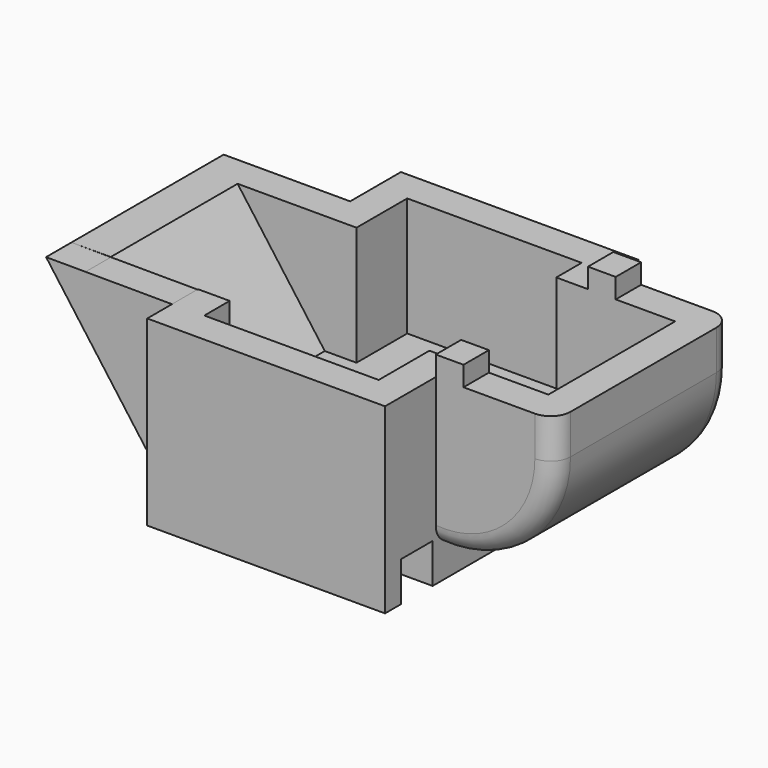
from build123d import *

# Parameters (mm, degrees)
F0_W      = 60
F0_H      = 80
F2_DEPTH  = 46
F1_W      = 30
F1_H      = 10
F3_DEPTH  = 10
F4_W      = 44
F4_H      = 64
F5_DEPTH  = 30
F6_W      = 8
F6_H      = 48
F7_DEPTH  = 30
F8_W      = 22
F8_H      = 30
F8_W_2    = 8
F9_DEPTH  = 8
F10_R     = 20
F12_DEPTH = 8
F14_DEPTH = 40
F15_R     = 5
F17_DEPTH = 8
F18_R     = 5
F19_W     = 7
F19_H     = 8
F20_DEPTH = 5
F21_W     = 22
F21_H     = 30
F21_W_2   = 8
F22_DEPTH = 8
F23_SIZE2 = 29.99999
F23_SIZE  = 21.99999
F25_DEPTH = 8
F27_DEPTH = 40
F29_DEPTH = 8


# Not quite as in the source:
# - a fillet or chamfer is up to 0.001 mm smaller than in the source, because OpenCascade refuses the exact size


with BuildPart() as f2:
    # F0 (on Top) → F2 (new body)
    with BuildSketch(Plane.XY):
        Rectangle(F0_W, F0_H)
    extrude(amount=F2_DEPTH)

    # F1 (on face) → F3 (cut)
    with BuildSketch(Plane.XY):
        with Locations((-15, 30)):
            Rectangle(F1_W, F1_H)
        with Locations((15, -30)):
            Rectangle(F1_W, F1_H)
    extrude(amount=F3_DEPTH, mode=Mode.SUBTRACT)

    # F4 (on face) → F5 (cut)
    with BuildSketch(Plane.XY.offset(46)):
        Rectangle(F4_W, F4_H)
    extrude(amount=-F5_DEPTH, mode=Mode.SUBTRACT)

    # F6 (on face) → F7 (cut, through all)
    with BuildSketch(Plane.XY.offset(46)):
        with Locations((-26, 0)):
            Rectangle(F6_W, F6_H)
        with Locations((26, 0)):
            Rectangle(F6_W, F6_H)
    extrude(amount=-F7_DEPTH, mode=Mode.SUBTRACT)

    # F8 (on face) → F9 (join)
    with BuildSketch(Plane(origin=(0, -24, 0), x_dir=(-1, 0, 0), z_dir=(0, 1, 0))):
        with Locations((-41, 31)):
            Rectangle(F8_W, F8_H)
        with Locations((-26, 31)):
            Rectangle(F8_W_2, F8_H)
    extrude(amount=F9_DEPTH)

    # F10
    f10_edges = [f2.edges().sort_by_distance(p)[0] for p in [
        (52, -20, 16),
    ]]
    fillet(f10_edges, radius=F10_R)

    # F11 (on face) → F12 (join, through all)
    with BuildSketch(Plane(origin=(0, -16, 0), x_dir=(-1, 0, 0), z_dir=(0, 1, 0))):
        with BuildLine():
            ThreePointArc((-58.1533936612, 46), (-59.5344785906, 41.08453427), (-60, 36))
            ThreePointArc((-60, 36), (-51.7989898732, 16.2010101268), (-32, 8))
            Line((-32, 8), (-32, 16))
            ThreePointArc((-32, 16), (-46.1421356237, 21.8578643763), (-52, 36))
            Line((-52, 36), (-52, 46))
            Line((-52, 46), (-58.1533936612, 46))
        make_face()
        with BuildLine():
            Line((-60, 46), (-60, 36))
            ThreePointArc((-60, 36), (-59.5344785906, 41.08453427), (-58.1533936612, 46))
            Line((-58.1533936612, 46), (-60, 46))
        make_face()
        with BuildLine():
            Line((-32, 16), (-32, 8))
            ThreePointArc((-32, 8), (-30.999360817, 8.0178856906), (-30, 8.0715199125))
            Line((-30, 8.0715199125), (-30, 16))
            Line((-30, 16), (-32, 16))
        make_face()
    extrude(amount=-F12_DEPTH)

    # F13 (on face) → F14 (join, through all)
    with BuildSketch(Plane(origin=(0, -16, 0), x_dir=(-1, 0, 0), z_dir=(0, 1, 0))):
        with BuildLine():
            ThreePointArc((-58.1533936612, 46), (-59.5344785906, 41.08453427), (-60, 36))
            Line((-60, 36), (-52, 36))
            Line((-52, 36), (-52, 46))
            Line((-52, 46), (-58.1533936612, 46))
        make_face()
        with BuildLine():
            Line((-60, 46), (-60, 36))
            ThreePointArc((-60, 36), (-59.5344785906, 41.08453427), (-58.1533936612, 46))
            Line((-58.1533936612, 46), (-60, 46))
        make_face()
        with BuildLine():
            Line((-52, 36), (-60, 36))
            ThreePointArc((-60, 36), (-51.7989898732, 16.2010101268), (-32, 8))
            Line((-32, 8), (-32, 16))
            ThreePointArc((-32, 16), (-46.1421356237, 21.8578643763), (-52, 36))
        make_face()
        with BuildLine():
            Line((-32, 16), (-32, 8))
            ThreePointArc((-32, 8), (-30.999360817, 8.0178856906), (-30, 8.0715199125))
            Line((-30, 8.0715199125), (-30, 16))
            Line((-30, 16), (-32, 16))
        make_face()
    extrude(amount=F14_DEPTH)

    # F15
    f15_edges = [f2.edges().sort_by_distance(p)[0] for p in [
        (51.078784, -24, 15.506098),
    ]]
    fillet(f15_edges, radius=F15_R)

    # F16 (on face) → F17 (join)
    with BuildSketch(Plane(origin=(0, 24, 0), x_dir=(-1, 0, 0), z_dir=(0, 1, 0))):
        with BuildLine():
            ThreePointArc((-30, 8.0715199125), (-30.999360817, 8.0178856906), (-32, 8))
            Line((-32, 8), (-30, 8))
            Line((-30, 8), (-30, 8.0715199125))
        make_face()
        with BuildLine():
            Line((-30, 16), (-32, 16))
            Line((-32, 16), (-32, 8))
            ThreePointArc((-32, 8), (-30.999360817, 8.0178856906), (-30, 8.0715199125))
            Line((-30, 8.0715199125), (-30, 16))
        make_face()
        with BuildLine():
            ThreePointArc((-32, 16), (-46.1421356237, 21.8578643763), (-52, 36))
            Line((-52, 36), (-60, 36))
            ThreePointArc((-60, 36), (-51.7989898732, 16.2010101268), (-32, 8))
            Line((-32, 8), (-32, 16))
        make_face()
        with BuildLine():
            Line((-60, 46), (-60, 36))
            ThreePointArc((-60, 36), (-59.5344785906, 41.08453427), (-58.1533936612, 46))
            Line((-58.1533936612, 46), (-60, 46))
        make_face()
        with BuildLine():
            Line((-60, 36), (-52, 36))
            Line((-52, 36), (-52, 46))
            Line((-52, 46), (-58.1533936612, 46))
            ThreePointArc((-58.1533936612, 46), (-59.5344785906, 41.08453427), (-60, 36))
        make_face()
        with BuildLine():
            ThreePointArc((-30, 16.1002512579), (-30.9987444988, 16.0250785378), (-32, 16))
            Line((-32, 16), (-30, 16))
            Line((-30, 16), (-30, 16.1002512579))
        make_face()
        with BuildLine():
            ThreePointArc((-49.3205080757, 46), (-51.3185165258, 41.1763809021), (-52, 36))
            ThreePointArc((-52, 36), (-46.1421356237, 21.8578643763), (-32, 16))
            ThreePointArc((-32, 16), (-30.9987444988, 16.0250785378), (-30, 16.1002512579))
            Line((-30, 16.1002512579), (-30, 46))
            Line((-30, 46), (-49.3205080757, 46))
        make_face()
        with BuildLine():
            Line((-52, 46), (-52, 36))
            ThreePointArc((-52, 36), (-51.3185165258, 41.1763809021), (-49.3205080757, 46))
            Line((-49.3205080757, 46), (-52, 46))
        make_face()
    extrude(amount=F17_DEPTH)

    # F18
    f18_edges = [f2.edges().sort_by_distance(p)[0] for p in [
        (51.79899, 32, 16.20101),
    ]]
    fillet(f18_edges, radius=F18_R)

    # F19 (on face) → F20 (join)
    with BuildSketch(Plane.XY.offset(46)):
        with Locations((33.5, 28)):
            Rectangle(F19_W, F19_H)
        with Locations((33.5, -20)):
            Rectangle(F19_W, F19_H)
    extrude(amount=F20_DEPTH)

    # F21 (on face) → F22 (join)
    with BuildSketch(Plane.XZ.offset(-24)):
        with Locations((-41, 31)):
            Rectangle(F21_W, F21_H)
        with Locations((-26, 31)):
            Rectangle(F21_W_2, F21_H)
    extrude(amount=F22_DEPTH)

    # F23 (size 22 and 30 in the source; OpenCascade refuses exactly that, so slightly less here)
    f23_edges = [f2.edges().sort_by_distance(p)[0] for p in [
        (-52, 20, 16),
    ]]
    f23_side = f2.faces().sort_by_distance((-41, 20, 16))[0]
    chamfer(f23_edges, length=F23_SIZE, length2=F23_SIZE2, reference=f23_side)

    # F24 (on face) → F25 (join)
    with BuildSketch(Plane.XZ.offset(-16)):
        Polygon((-30, 16), (-52, 46), (-61.9205734601, 46), (-30, 2.4719452816), align=None)
    extrude(amount=-F25_DEPTH)

    # F26 (on face) → F27 (join, through all)
    with BuildSketch(Plane.XZ.offset(-16)):
        Polygon((-61.9205734601, 46), (-30, 2.4719452816), (-30, 16), (-52, 46), align=None)
    extrude(amount=F27_DEPTH)

    # F28 (on face) → F29 (join)
    with BuildSketch(Plane.XZ.offset(24)):
        Polygon((-51.9714293201, 45.961039982), (-30, 16), (-30, 45.8750016987), align=None)
        Polygon((-61.9205734601, 46), (-30, 2.4719452816), (-30, 16), (-51.9714293201, 45.961039982), align=None)
    extrude(amount=F29_DEPTH)


solid = f2.part
